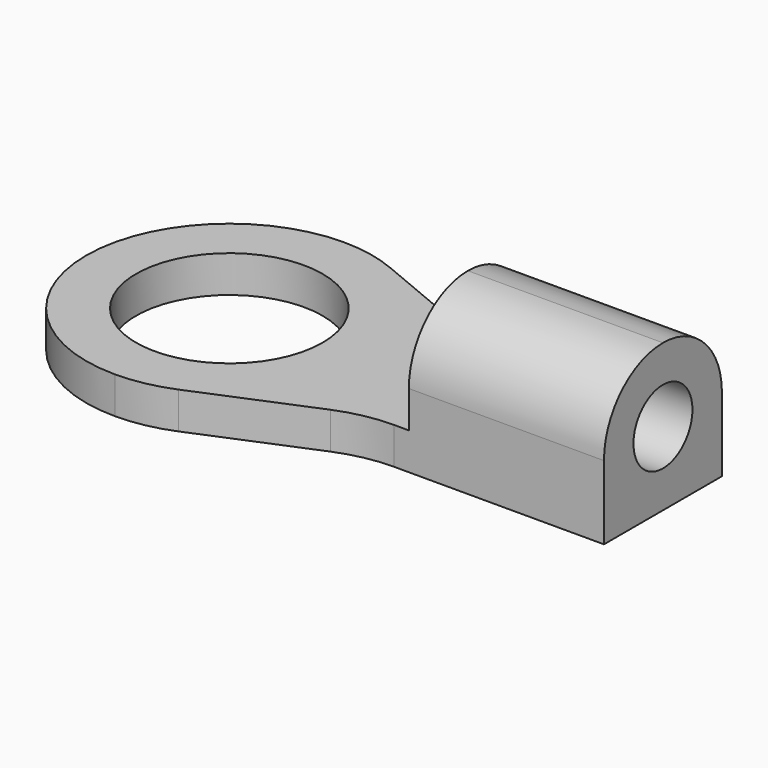
from build123d import *

# Parameters (mm, degrees)
F0_R     = 2.15
F1_DEPTH = 0.85
F2_W     = 4.5
F2_H     = 3.4
F3_DEPTH = 2.55
F4_R     = 1.69999
F5_R     = 0.85
F6_DEPTH = 25


# Not quite as in the source:
# - a fillet or chamfer is up to 0.001 mm smaller than in the source, because OpenCascade refuses the exact size


with BuildPart() as f1:
    # F0 (on Top) → F1 (new body)
    with BuildSketch(Plane.XY):
        with BuildLine():
            Line((8.46, 1.6), (13.3, 1.6))
            Line((13.3, 1.6), (13.3, 5))
            Line((13.3, 5), (8.46, 5))
            ThreePointArc((8.46, 5), (7.812816754, 5.0640837702), (7.1907692308, 5.2538461538))
            Line((7.1907692308, 5.2538461538), (4.5692307692, 6.3461538462))
            ThreePointArc((4.5692307692, 6.3461538462), (3.947183246, 6.5359162298), (3.3, 6.6))
            ThreePointArc((3.3, 6.6), (0.9665476221, 5.6334523779), (0, 3.3))
            ThreePointArc((0, 3.3), (0.9665476221, 0.9665476221), (3.3, 0))
            ThreePointArc((3.3, 0), (3.947183246, 0.0640837702), (4.5692307692, 0.2538461538))
            Line((4.5692307692, 0.2538461538), (7.1907692308, 1.3461538462))
            ThreePointArc((7.1907692308, 1.3461538462), (7.812816754, 1.5359162298), (8.46, 1.6))
        make_face()
        with Locations((3.3, 3.3)):
            Circle(F0_R, mode=Mode.SUBTRACT)
    extrude(amount=F1_DEPTH)

    # F2 (on face) → F3 (join)
    with BuildSketch(Plane.XY.offset(0.85)):
        with Locations((11.05, 3.3)):
            Rectangle(F2_W, F2_H)
    extrude(amount=F3_DEPTH)

    # F4 (radius 1.7 in the source; OpenCascade refuses exactly that, so slightly less here)
    f4_edges = [f1.edges().sort_by_distance(p)[0] for p in [
        (11.05, 5, 3.4),
        (11.05, 1.6, 3.4),
    ]]
    fillet(f4_edges, radius=F4_R)

    # F5 (on face) → F6 (cut)
    with BuildSketch(Plane.YZ.offset(13.3)):
        with Locations((3.3, 1.7)):
            Circle(F5_R)
    extrude(amount=-F6_DEPTH, mode=Mode.SUBTRACT)


solid = f1.part
